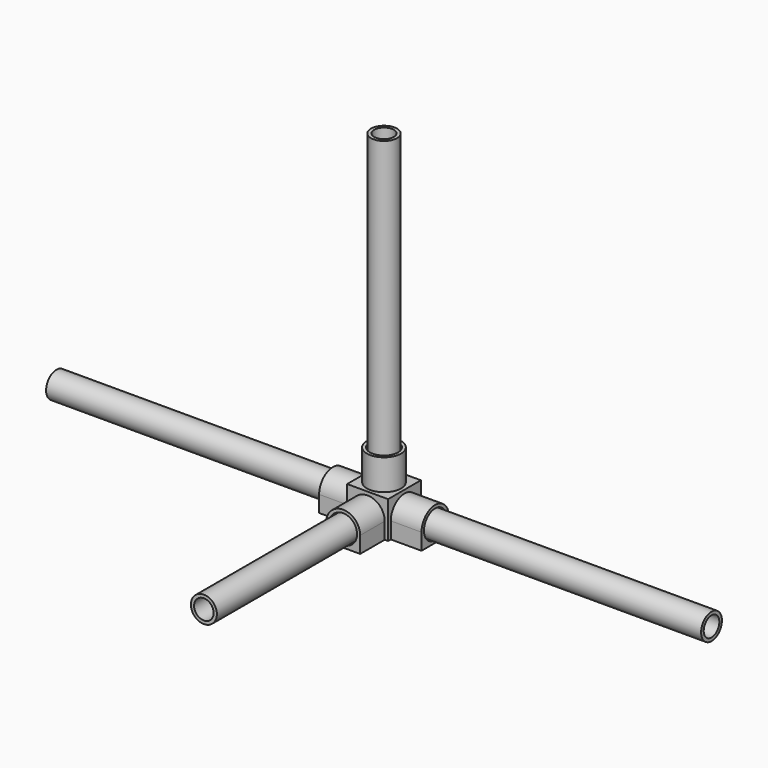
from build123d import *

# Parameters (mm, degrees)
F0_W      = 40
F0_H      = 40
F1_DEPTH  = 20
F2_R      = 13.7
F2_R_2    = 12.7
F2_R_3    = 9.55
F3_DEPTH  = 3
F4_DEPTH  = 200
F5_DEPTH  = 3
F2_R_4    = 16.7
F6_DEPTH  = 30
F7_R      = 13.7
F7_R_2    = 12.7
F7_R_3    = 9.55
F8_DEPTH  = 3
F9_DEPTH  = 300
F7_R_4    = 16.7
F10_DEPTH = 30
F11_R     = 13.7
F11_R_2   = 12.7
F11_R_3   = 9.55
F12_DEPTH = 3
F13_DEPTH = 300
F11_R_4   = 16.7
F14_DEPTH = 30
F15_R     = 13.7
F15_R_2   = 12.7
F15_R_3   = 9.55
F16_DEPTH = 3
F17_DEPTH = 300
F15_R_4   = 16.7
F18_DEPTH = 30
F21_DEPTH = 30
F22_DEPTH = 30
F24_DEPTH = 30
F25_DEPTH = 4


with BuildPart() as f1:
    # F0 (on Front) → F1 (new body, symmetric)
    with BuildSketch(Plane.XZ):
        Rectangle(F0_W, F0_H)
    extrude(amount=F1_DEPTH, both=True)

    # F2 (on face) → F3 (cut)
    with BuildSketch(Plane.XZ.offset(20)):
        Circle(F2_R)
        Circle(F2_R_2, mode=Mode.SUBTRACT)
        Circle(F2_R_2)
        Circle(F2_R_3, mode=Mode.SUBTRACT)
        Circle(F2_R_3)
    extrude(amount=-F3_DEPTH, mode=Mode.SUBTRACT)

    # F2 (on face) → F6 (join)
    with BuildSketch(Plane.XZ.offset(20)):
        Circle(F2_R_4)
        Circle(F2_R, mode=Mode.SUBTRACT)
    extrude(amount=F6_DEPTH)

    # F7 (on face) → F8 (cut)
    with BuildSketch(Plane.YZ.offset(20)):
        Circle(F7_R)
        Circle(F7_R_2, mode=Mode.SUBTRACT)
        Circle(F7_R_2)
        Circle(F7_R_3, mode=Mode.SUBTRACT)
        Circle(F7_R_3)
    extrude(amount=-F8_DEPTH, mode=Mode.SUBTRACT)

    # F7 (on face) → F10 (join)
    with BuildSketch(Plane.YZ.offset(20)):
        Circle(F7_R_4)
        Circle(F7_R, mode=Mode.SUBTRACT)
    extrude(amount=F10_DEPTH)

    # F11 (on face) → F12 (cut)
    with BuildSketch(Plane(origin=(-20, 0, 0), x_dir=(0, -1, 0), z_dir=(-1, 0, 0))):
        Circle(F11_R)
        Circle(F11_R_2, mode=Mode.SUBTRACT)
        Circle(F11_R_2)
        Circle(F11_R_3, mode=Mode.SUBTRACT)
        Circle(F11_R_3)
    extrude(amount=-F12_DEPTH, mode=Mode.SUBTRACT)

    # F11 (on face) → F14 (join)
    with BuildSketch(Plane(origin=(-20, 0, 0), x_dir=(0, -1, 0), z_dir=(-1, 0, 0))):
        Circle(F11_R_4)
        Circle(F11_R, mode=Mode.SUBTRACT)
    extrude(amount=F14_DEPTH)

    # F15 (on face) → F16 (cut)
    with BuildSketch(Plane.XY.offset(20)):
        Circle(F15_R)
        Circle(F15_R_2, mode=Mode.SUBTRACT)
        Circle(F15_R_2)
        Circle(F15_R_3, mode=Mode.SUBTRACT)
        Circle(F15_R_3)
    extrude(amount=-F16_DEPTH, mode=Mode.SUBTRACT)

    # F15 (on face) → F18 (join)
    with BuildSketch(Plane.XY.offset(20)):
        Circle(F15_R_4)
        Circle(F15_R, mode=Mode.SUBTRACT)
    extrude(amount=F18_DEPTH)

    # F19 (on face) → F21 (join, through all)
    with BuildSketch(Plane(origin=(-20, 0, 0), x_dir=(0, -1, 0), z_dir=(-1, 0, 0))):
        with BuildLine():
            ThreePointArc((16.7, 0), (0, -16.7), (-16.7, 0))
            Line((-16.7, 0), (-16.7, -20))
            Line((-16.7, -20), (16.7, -20))
            Line((16.7, -20), (16.7, 0))
        make_face()
    extrude(amount=F21_DEPTH)

    # F20 (on face) → F22 (join, through all)
    with BuildSketch(Plane.XZ.offset(20)):
        with BuildLine():
            ThreePointArc((16.7, 0), (0, -16.7), (-16.7, 0))
            Line((-16.7, 0), (-16.7, -20))
            Line((-16.7, -20), (16.7, -20))
            Line((16.7, -20), (16.7, 0))
        make_face()
    extrude(amount=F22_DEPTH)

    # F23 (on face) → F24 (join, through all)
    with BuildSketch(Plane.YZ.offset(20)):
        with BuildLine():
            ThreePointArc((16.7, 0), (0, -16.7), (-16.7, 0))
            Line((-16.7, 0), (-16.7, -20))
            Line((-16.7, -20), (16.7, -20))
            Line((16.7, -20), (16.7, 0))
        make_face()
    extrude(amount=F24_DEPTH)

    # F25 (cut): a face of the model
    f25_faces = [f1.faces().sort_by_distance(p)[0] for p in [
        (0, -7.6139817629, -20),
    ]]
    extrude(f25_faces, amount=-F25_DEPTH, mode=Mode.SUBTRACT)


with BuildPart() as f4:
    # F2 (on face) → F4 (new body)
    with BuildSketch(Plane.XZ.offset(20)):
        Circle(F2_R_2)
        Circle(F2_R_3, mode=Mode.SUBTRACT)
    extrude(amount=F4_DEPTH)

    # F5 (add): a face of the model
    f5_faces = [f4.faces().sort_by_distance(p)[0] for p in [
        (-12.3407897552, -20, 0),
    ]]
    extrude(f5_faces, amount=F5_DEPTH)


with BuildPart() as f9:
    # F7 (on face) → F9 (new body)
    with BuildSketch(Plane.YZ.offset(20)):
        Circle(F7_R_2)
        Circle(F7_R_3, mode=Mode.SUBTRACT)
    extrude(amount=F9_DEPTH)


with BuildPart() as f13:
    # F11 (on face) → F13 (new body)
    with BuildSketch(Plane(origin=(-20, 0, 0), x_dir=(0, -1, 0), z_dir=(-1, 0, 0))):
        Circle(F11_R_2)
        Circle(F11_R_3, mode=Mode.SUBTRACT)
    extrude(amount=F13_DEPTH)


with BuildPart() as f17:
    # F15 (on face) → F17 (new body)
    with BuildSketch(Plane.XY.offset(20)):
        Circle(F15_R_2)
        Circle(F15_R_3, mode=Mode.SUBTRACT)
    extrude(amount=F17_DEPTH)


with BuildPart() as f26_1:
    # F26: copy of F1
    add(f1.part)


solid = Compound([f1.part, f4.part, f9.part, f13.part, f17.part, f26_1.part])
